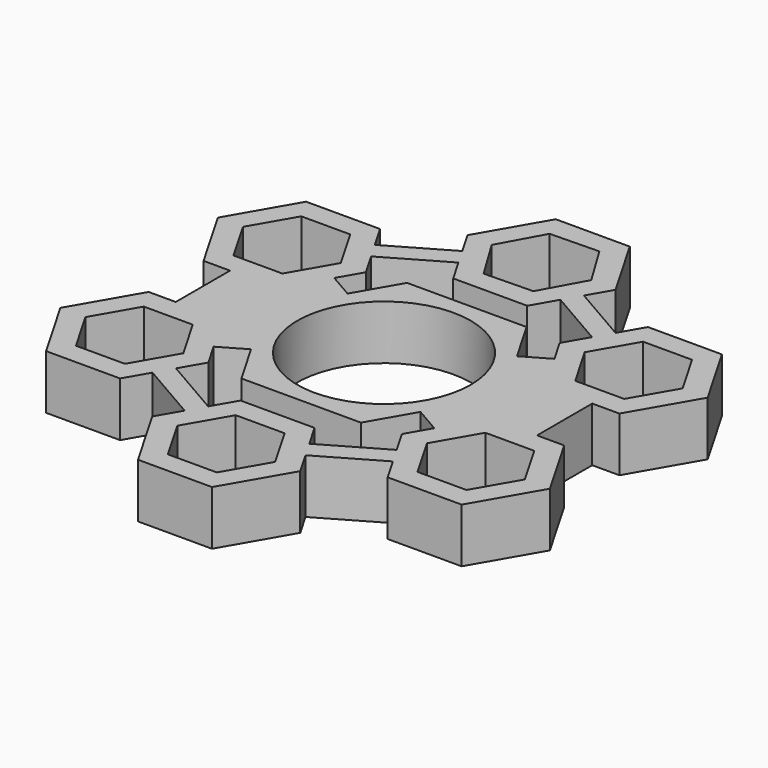
from build123d import *

# Parameters (mm, degrees)
F0_W     = 2.54
F0_H     = 8.7372876405
F0_H_2   = 8.89
F1_DEPTH = 6.9977
F2_R     = 11.176
F3_DEPTH = 6.9977


with BuildPart() as f1:
    # F0 (on Top) → F1 (new body)
    with BuildSketch(Plane.XY):
        Polygon((-11.6335226281, 5.2501477372), (-10.3635226281, 7.4498522628), (-14.0807527651, 9.595996083), (-15.3507527651, 7.3962915574), align=None)
        Polygon((-14.6646968374, 0), (-11.6335226281, 5.2501477372), (-15.3507527651, 7.3962915574), (-17.1428502621, 4.2922876405), (-20.7270452561, 4.2922876405), (-20.7270452561, -4.445), (-17.231018784, -4.445), (-15.4830055479, -7.4726477372), (-11.6335226281, -5.2501477372), align=None)
        Polygon((-15.3507527651, 7.3962915574), (-14.0807527651, 9.595996083), (-12.3768237899, 12.5472876405), (-14.124837026, 15.5749353777), (-14.2130055479, 15.7276477372), (-15.394837026, 17.7746399033), (-17.1428502621, 20.8022876405), (-26.6749032064, 20.8022876405), (-31.4409296786, 12.5472876405), (-26.6749032064, 4.2922876405), (-23.2670452561, 4.2922876405), (-20.7270452561, 4.2922876405), (-17.1428502621, 4.2922876405), align=None)
        Polygon((-18.7559669142, 18.0082876405), (-15.6030570942, 12.5472876405), (-18.7559669142, 7.0862876405), (-25.0617865543, 7.0862876405), (-28.2146963743, 12.5472876405), (-25.0617865543, 18.0082876405), align=None, mode=Mode.SUBTRACT)
        Polygon((14.2130055479, 9.6723522628), (10.3635226281, 7.4498522628), (11.6335226281, 5.2501477372), (15.4830055479, 7.4726477372), align=None)
        Polygon((-10.3635226281, -7.4498522628), (-11.6335226281, -5.2501477372), (-15.4830055479, -7.4726477372), (-14.2130055479, -9.6723522628), align=None)
        Polygon((-14.2130055479, 15.7276477372), (-14.124837026, 15.5749353777), (-6.4258711864, 20.0199353777), (-7.6958711864, 22.2196399033), (-15.394837026, 17.7746399033), align=None)
        Polygon((15.4830055479, 7.4726477372), (11.6335226281, 5.2501477372), (14.6646968374, 0), (11.6335226281, -5.2501477372), (15.4830055479, -7.4726477372), (17.231018784, -4.445), (20.7270452561, -4.445), (20.7270452561, 4.445), (17.231018784, 4.445), align=None)
        Polygon((12.4649923118, 12.7), (14.2130055479, 9.6723522628), (15.4830055479, 7.4726477372), (17.231018784, 4.445), (20.7270452561, 4.445), (23.2670452561, 4.445), (26.7630717283, 4.445), (31.5290982004, 12.7), (26.7630717283, 20.955), (17.231018784, 20.955), (15.4830055479, 17.9273522628), (14.2130055479, 15.7276477372), align=None)
        Polygon((25.1499550762, 7.239), (18.8441354361, 7.239), (15.691225616, 12.7), (18.8441354361, 18.161), (25.1499550762, 18.161), (28.3028648962, 12.7), align=None, mode=Mode.SUBTRACT)
        Polygon((-14.2130055479, -9.6723522628), (-15.4830055479, -7.4726477372), (-17.231018784, -4.445), (-20.7270452561, -4.445), (-23.2670452561, -4.445), (-26.7630717283, -4.445), (-31.5290982004, -12.7), (-26.7630717283, -20.955), (-17.231018784, -20.955), (-15.4830055479, -17.9273522628), (-14.2130055479, -15.7276477372), (-12.4649923118, -12.7), align=None)
        Polygon((-25.1499550762, -7.239), (-18.8441354361, -7.239), (-15.691225616, -12.7), (-18.8441354361, -18.161), (-25.1499550762, -18.161), (-28.3028648962, -12.7), align=None, mode=Mode.SUBTRACT)
        with Locations((-21.9970452561, -0.0763561798)):
            Rectangle(F0_W, F0_H)
        Polygon((-7.6958711864, 22.2196399033), (-6.4258711864, 20.0199353777), (-4.6778579503, 16.9922876405), (-1.27, 16.9922876405), (1.27, 16.9922876405), (4.854194994, 16.9922876405), (6.6462924911, 20.0962915574), (7.9162924911, 22.295996083), (9.6202214662, 25.2472876405), (4.854194994, 33.5022876405), (-4.6778579503, 33.5022876405), (-9.4438844224, 25.2472876405), align=None)
        Polygon((6.3924737908, 25.3854774003), (3.3599969989, 19.8566940043), (-2.94430827, 19.7185042444), (-6.216136747, 25.1090978806), (-3.1836599552, 30.6378812766), (3.1206453137, 30.7760710365), align=None, mode=Mode.SUBTRACT)
        Polygon((15.4830055479, -7.4726477372), (11.6335226281, -5.2501477372), (10.3635226281, -7.4498522628), (14.2130055479, -9.6723522628), align=None)
        Polygon((6.6462924911, 20.0962915574), (14.2130055479, 15.7276477372), (15.4830055479, 17.9273522628), (7.9162924911, 22.295996083), align=None)
        Polygon((17.231018784, -4.445), (15.4830055479, -7.4726477372), (14.2130055479, -9.6723522628), (12.4649923118, -12.7), (14.2130055479, -15.7276477372), (15.4830055479, -17.9273522628), (17.231018784, -20.955), (26.7630717283, -20.955), (31.5290982004, -12.7), (26.7630717283, -4.445), (23.2670452561, -4.445), (20.7270452561, -4.445), align=None)
        Polygon((18.8441354361, -18.161), (15.691225616, -12.7), (18.8441354361, -7.239), (25.1499550762, -7.239), (28.3028648962, -12.7), (25.1499550762, -18.161), align=None, mode=Mode.SUBTRACT)
        with Locations((21.9970452561, 0)):
            Rectangle(F0_W, F0_H_2)
        Polygon((-6.5140397082, -20.1726477372), (-14.2130055479, -15.7276477372), (-15.4830055479, -17.9273522628), (-7.7840397082, -22.3723522628), align=None)
        Polygon((-4.7660264722, -17.145), (-6.5140397082, -20.1726477372), (-7.7840397082, -22.3723522628), (-9.5320529443, -25.4), (-4.7660264722, -33.655), (4.7660264722, -33.655), (9.5320529443, -25.4), (7.7840397082, -22.3723522628), (6.5140397082, -20.1726477372), (4.7660264722, -17.145), (1.27, -17.145), (-1.27, -17.145), align=None)
        Polygon((-6.3058196401, -25.4), (-3.15290982, -19.939), (3.15290982, -19.939), (6.3058196401, -25.4), (3.15290982, -30.861), (-3.15290982, -30.861), align=None, mode=Mode.SUBTRACT)
        Polygon((15.4830055479, -17.9273522628), (14.2130055479, -15.7276477372), (6.5140397082, -20.1726477372), (7.7840397082, -22.3723522628), align=None)
    extrude(amount=F1_DEPTH)

    # F2 (on Top) → F3 (join)
    with BuildSketch(Plane.XY):
        Polygon((7.6989658396, 13.335), (-7.6989658396, 13.335), (-15.3979316793, 0), (-7.6989658396, -13.335), (7.6989658396, -13.335), (15.3979316793, 0), align=None)
        Circle(F2_R, mode=Mode.SUBTRACT)
    extrude(amount=F3_DEPTH)


solid = f1.part
